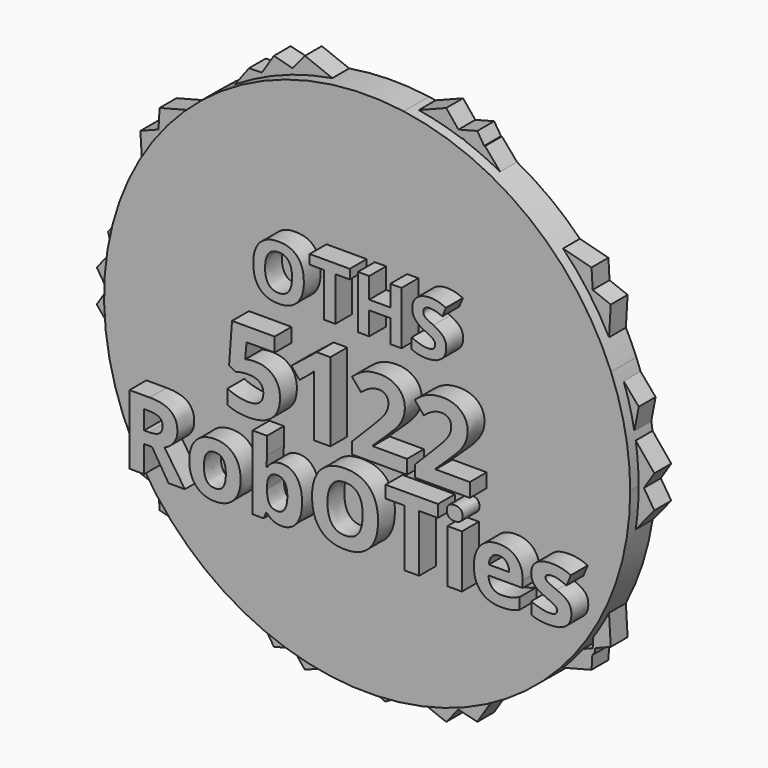
from build123d import *

# Parameters (mm, degrees)
F1_DEPTH       = 7.62
F3_DEPTH       = 5.08
F4_TEXT_SIZE   = 17.9359663485
F4_TEXT_SIZE_2 = 26.5140358048
F4_TEXT_SIZE_3 = 23.3947377031
F5_DEPTH       = 5.08
F6_DEPTH       = 12.7


# Not quite as in the source:
# - Text() gives the source's letters only with a copy of the font that has no kerning and outlines rounded to 1/6400 em; it was checked with that copy


with BuildPart() as f1:
    # F0 (on Front) → F1 (new body)
    with BuildSketch(Plane.XZ):
        with BuildLine():
            ThreePointArc((-8.8088285315, -62.7875043569), (23.7650828926, -58.7799880791), (49.9711595476, -39.0224214643))
            Line((49.9711595476, -39.0224214643), (-8.8088285315, -62.7875043569))
        make_face()
        Polygon((-8.8088285315, -62.7875043569), (49.9711595476, -39.0224214643), (58.7799880791, 23.7650828926), (8.8088285315, 62.7875043569), (-49.9711595476, 39.0224214643), (-58.7799880791, -23.7650828926), align=None)
        with BuildLine():
            Line((58.7799880791, 23.7650828926), (49.9711595476, -39.0224214643))
            ThreePointArc((49.9711595476, -39.0224214643), (59.9506394201, -20.6346067707), (63.4024144924, 0))
            ThreePointArc((63.4024144924, 0), (62.2360800963, 12.1052260495), (58.7799880791, 23.7650828926))
        make_face()
        with BuildLine():
            ThreePointArc((-58.7799880791, -23.7650828926), (-39.0224214643, -49.9711595476), (-8.8088285315, -62.7875043569))
            Line((-8.8088285315, -62.7875043569), (-58.7799880791, -23.7650828926))
        make_face()
        with BuildLine():
            Line((8.8088285315, 62.7875043569), (58.7799880791, 23.7650828926))
            ThreePointArc((58.7799880791, 23.7650828926), (39.0224214643, 49.9711595476), (8.8088285315, 62.7875043569))
        make_face()
        with BuildLine():
            ThreePointArc((-49.9711595476, 39.0224214643), (-62.7875043569, 8.8088285315), (-58.7799880791, -23.7650828926))
            Line((-58.7799880791, -23.7650828926), (-49.9711595476, 39.0224214643))
        make_face()
        with BuildLine():
            Line((-49.9711595476, 39.0224214643), (8.8088285315, 62.7875043569))
            ThreePointArc((8.8088285315, 62.7875043569), (-23.7650828926, 58.7799880791), (-49.9711595476, 39.0224214643))
        make_face()
    extrude(amount=F1_DEPTH)

    # F2 (on Front) → F3 (join)
    with BuildSketch(Plane.XZ):
        Polygon((57.0870039693, -16.2666344092), (67.1984978823, -3.9355448567), (64.6769401119, 0), (58.2957219965, -9.9595458127), align=None)
        Polygon((55.8744273316, -22.5938572285), (57.0870039693, -16.2666344092), (55.6094006656, -18.068589572), align=None)
        Polygon((55.6094006656, -18.068589572), (57.0870039693, -16.2666344092), (58.2957219965, -9.9595458127), (55.3992459704, -14.480247841), align=None)
        Polygon((58.2957219965, -9.9595458127), (64.6769401119, 0), (61.2341795578, 5.373320711), align=None)
        Polygon((61.2341795578, 5.373320711), (64.6769401119, 0), (67.1984978823, 3.9355448567), (62.1407074463, 10.103581681), align=None)
        Polygon((55.8744273316, -22.5938572285), (55.6094006656, -18.068589572), (53.3302075961, -20.8480931834), (52.3247436947, -38.0161515612), (52.9669441343, -37.7650995737), align=None)
        Polygon((56.6779820097, -36.3143633602), (55.8744273316, -22.5938572285), (52.9669441343, -37.7650995737), align=None)
        Polygon((55.3992459704, 14.480247841), (61.2341795578, 5.373320711), (62.1407074463, 10.103581681), (55.6094006656, 18.068589572), align=None)
        Polygon((52.7120965601, -39.0948937797), (52.9669441343, -37.7650995737), (52.3247436947, -38.0161515612), (52.2472597228, -39.3391720605), align=None)
        Polygon((55.6094006656, 18.068589572), (62.1407074463, 10.103581681), (63.4310734005, 16.8367090212), (56.0424797884, 25.4633131937), align=None)
        Polygon((52.2472597228, -39.3391720605), (52.3247436947, -38.0161515612), (36.3076553351, -44.2776263556), (34.3684997054, -47.3041816282), (39.7844205524, -45.8885689284), align=None)
        Polygon((53.3302075961, 20.8480931834), (55.6094006656, 18.068589572), (56.0424797884, 25.4633131937), (52.8409983588, 29.2012252388), align=None)
        Polygon((52.0514715567, -42.6822087026), (52.2472597228, -39.3391720605), (39.7844205524, -45.8885689284), align=None)
        Polygon((52.8409983588, 29.2012252388), (56.0424797884, 25.4633131937), (56.6779820097, 36.3143633602), (52.3247436947, 38.0161515612), align=None)
        Polygon((34.3684997054, -47.3041816282), (30.8908425472, -48.2131712123), (27.5059662196, -52.3410689769), (32.9866729199, -49.4608806982), align=None)
        Polygon((39.7844205524, -45.8885689284), (34.3684997054, -47.3041816282), (32.9866729199, -49.4608806982), align=None)
        Polygon((34.3684997054, 47.3041816282), (36.3076553351, 44.2776263556), (41.7506674371, 42.1498187094), (38.191967079, 46.3048042141), align=None)
        Polygon((41.7506674371, 42.1498187094), (52.8409983588, 29.2012252388), (52.3247436947, 38.0161515612), align=None)
        Polygon((32.9866729199, -49.4608806982), (27.5059662196, -52.3410689769), (19.9862736387, -61.5114253474), (24.5084034232, -62.6934190533), align=None)
        Polygon((19.9862736387, -61.5114253474), (27.5059662196, -52.3410689769), (13.3543091922, -59.7779633269), align=None)
        Polygon((13.3543091922, -59.7779633269), (3.3477744136, -57.1624565436), (0, -58.4711841124), (9.0837021311, -62.0222272644), align=None)
        Polygon((30.8908425472, 48.2131712123), (34.3684997054, 47.3041816282), (26.1810818752, 60.0827705265), (21.2981716078, 59.9115498513), align=None)
        Polygon((26.1810818752, 60.0827705265), (34.3684997054, 47.3041816282), (38.191967079, 46.3048042141), (26.3851582123, 60.0899265228), align=None)
        Polygon((38.191967079, 46.3048042141), (41.7506674371, 42.1498187094), (52.3247436947, 38.0161515612), (52.0514715567, 42.6822087026), align=None)
        Polygon((17.022552261, -65.125719539), (19.9862736387, -61.5114253474), (13.3543091922, -59.7779633269), (9.0837021311, -62.0222272644), align=None)
        Polygon((-7.3567150808, -61.3471054418), (0, -58.4711841124), (-3.3477744136, -57.1624565436), (-11.8348123178, -59.3807974278), align=None)
        Polygon((9.0837021311, -62.0222272644), (0, -58.4711841124), (-7.3567150808, -61.3471054418), (2.2998358791, -65.587244174), align=None)
        Polygon((21.2981716078, 59.9115498513), (26.1810818752, 60.0827705265), (24.5084034232, 62.6934190533), (19.9862736387, 61.5114253474), align=None)
        Polygon((12.713752442, 59.6105346852), (21.2981716078, 59.9115498513), (19.9862736387, 61.5114253474), align=None)
        Polygon((0, 58.4711841124), (3.3477744136, 57.1624565436), (12.713752442, 59.6105346852), (1.9489135172, 59.2330624633), align=None)
        Polygon((-17.022552261, -65.125719539), (-7.3567150808, -61.3471054418), (-11.8348123178, -59.3807974278), (-19.9862736387, -61.5114253474), align=None)
        Polygon((-27.3027283004, -52.588920086), (-30.8908425472, -48.2131712123), (-34.3684997054, -47.3041816282), (-32.4230015154, -50.3406361109), align=None)
        Polygon((-19.9862736387, -61.5114253474), (-11.8348123178, -59.3807974278), (-27.3027283004, -52.588920086), align=None)
        Polygon((12.713752442, 59.6105346852), (19.9862736387, 61.5114253474), (17.022552261, 65.125719539), (1.9489135172, 59.2330624633), align=None)
        Polygon((-9.7060363636, 58.8243782406), (-3.3477744136, 57.1624565436), (0, 58.4711841124), (-1.628064531, 59.1076346829), align=None)
        Polygon((-1.628064531, 59.1076346829), (0, 58.4711841124), (1.9489135172, 59.2330624633), align=None)
        Polygon((-34.3684997054, -47.3041816282), (-36.3076553351, -44.2776263556), (-50.9416036357, -38.5568551162), (-49.844248127, -42.6910619693), (-46.6477166179, -44.0946414788), align=None)
        Polygon((-32.4230015154, -50.3406361109), (-34.3684997054, -47.3041816282), (-46.6477166179, -44.0946414788), align=None)
        Polygon((-19.9862736387, -61.5114253474), (-27.3027283004, -52.588920086), (-32.4230015154, -50.3406361109), (-24.5084034232, -62.6934190533), align=None)
        Polygon((-34.3684997054, 47.3041816282), (-30.8908425472, 48.2131712123), (-22.5592271175, 58.3736773516), (-27.3845306043, 58.204476675), align=None)
        Polygon((-22.5592271175, 58.3736773516), (-9.7060363636, 58.8243782406), (-19.9862736387, 61.5114253474), align=None)
        Polygon((-19.9862736387, 61.5114253474), (-9.7060363636, 58.8243782406), (-1.628064531, 59.1076346829), (-17.022552261, 65.125719539), align=None)
        Polygon((-49.844248127, -42.6910619693), (-50.9416036357, -38.5568551162), (-52.3247436947, -38.0161515612), (-52.0514715567, -42.6822087026), (-46.6477166179, -44.0946414788), align=None)
        Polygon((-52.3247436947, -38.0161515612), (-50.9416036357, -38.5568551162), (-52.6756911407, -32.0238069016), align=None)
        Polygon((-52.6756911407, -32.0238069016), (-53.3302075961, -20.8480931834), (-55.6094006656, -18.068589572), (-55.7486701258, -20.4465826755), align=None)
        Polygon((-36.3076553351, 44.2776263556), (-34.3684997054, 47.3041816282), (-39.5331397339, 45.9542486767), (-42.6014329749, 41.8172334822), align=None)
        Polygon((-39.5331397339, 45.9542486767), (-34.3684997054, 47.3041816282), (-27.3845306043, 58.204476675), (-30.529319269, 58.0942037417), align=None)
        Polygon((-27.3845306043, 58.204476675), (-22.5592271175, 58.3736773516), (-19.9862736387, 61.5114253474), (-24.5084034232, 62.6934190533), align=None)
        Polygon((-56.6779820097, -36.3143633602), (-52.3247436947, -38.0161515612), (-52.6756911407, -32.0238069016), (-55.7486701258, -20.4465826755), align=None)
        Polygon((-56.748638321, -16.679275424), (-55.6094006656, -18.068589572), (-55.3992459704, -14.480247841), (-58.6995909957, -9.3292034976), align=None)
        Polygon((-55.7486701258, -20.4465826755), (-55.6094006656, -18.068589572), (-56.748638321, -16.679275424), align=None)
        Polygon((-42.6014329749, 41.8172334822), (-39.5331397339, 45.9542486767), (-52.0514715567, 42.6822087026), (-52.3247436947, 38.0161515612), align=None)
        Polygon((-52.9166744209, 27.9090743705), (-42.6014329749, 41.8172334822), (-52.3247436947, 38.0161515612), align=None)
        Polygon((-55.6094006656, 18.068589572), (-53.3302075961, 20.8480931834), (-52.9166744209, 27.9090743705), (-55.9464698513, 23.8239662184), align=None)
        Polygon((-67.1984978823, -3.9355448567), (-56.748638321, -16.679275424), (-58.6995909957, -9.3292034976), (-64.6769401119, 0), align=None)
        Polygon((-62.201421736, 3.8636884414), (-55.3992459704, 14.480247841), (-55.6094006656, 18.068589572), (-63.4378216931, 8.5217351136), align=None)
        Polygon((-64.6769401119, 0), (-58.6995909957, -9.3292034976), (-62.201421736, 3.8636884414), align=None)
        Polygon((-52.9166744209, 27.9090743705), (-52.3247436947, 38.0161515612), (-56.6779820097, 36.3143633602), (-55.9464698513, 23.8239662184), align=None)
        Polygon((-63.4378216931, 8.5217351136), (-55.6094006656, 18.068589572), (-55.9464698513, 23.8239662184), (-64.4545966561, 12.3523606373), align=None)
        Polygon((-64.6769401119, 0), (-62.201421736, 3.8636884414), (-63.4378216931, 8.5217351136), (-67.1984978823, 3.9355448567), align=None)
    extrude(amount=F3_DEPTH)

    # F4 (on Front) → F5 (join)
    with BuildSketch(Plane.XZ):
        with Locations((-24.4241058826, 15.721263364)):
            Text('OTHS', F4_TEXT_SIZE, font='Open Sans', font_style=FontStyle.BOLD, text_align=(TextAlign.LEFT, TextAlign.BOTTOM))
        with Locations((-30.8810491115, -10.6680011377)):
            Text('5122', F4_TEXT_SIZE_2, font='Open Sans', font_style=FontStyle.BOLD, text_align=(TextAlign.LEFT, TextAlign.BOTTOM))
        with Locations((-55.3051717579, -31.161788851)):
            Text('RobOTies', F4_TEXT_SIZE_3, font='Open Sans', font_style=FontStyle.BOLD, text_align=(TextAlign.LEFT, TextAlign.BOTTOM))
    extrude(amount=F5_DEPTH)

    # F4 (on Front) → F6 (join)
    with BuildSketch(Plane.XZ):
        with Locations((-24.4241058826, 15.721263364)):
            Text('OTHS', F4_TEXT_SIZE, font='Open Sans', font_style=FontStyle.BOLD, text_align=(TextAlign.LEFT, TextAlign.BOTTOM))
        with Locations((-30.8810491115, -10.6680011377)):
            Text('5122', F4_TEXT_SIZE_2, font='Open Sans', font_style=FontStyle.BOLD, text_align=(TextAlign.LEFT, TextAlign.BOTTOM))
        with Locations((-55.3051717579, -31.161788851)):
            Text('RobOTies', F4_TEXT_SIZE_3, font='Open Sans', font_style=FontStyle.BOLD, text_align=(TextAlign.LEFT, TextAlign.BOTTOM))
    extrude(amount=F6_DEPTH)


solid = f1.part
